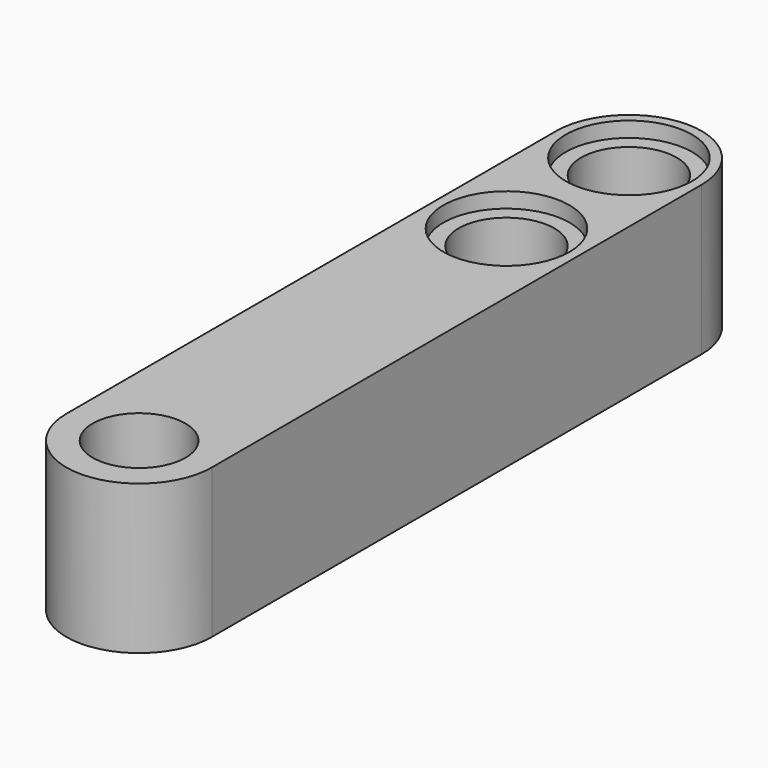
from build123d import *

# Parameters (mm, degrees)
F0_R      = 2.5
F1_DEPTH  = 7.8
F2_R      = 3.3
F3_DEPTH  = 0.8
F4_R      = 3.3
F5_DEPTH  = 0.8
F6_R      = 2.425
F7_DEPTH  = 2.8
F8_R      = 1.75
F9_DEPTH  = 4
F10_R     = 1.15
F11_DEPTH = 5.001
F12_R     = 0.59999
F13_R     = 0.4


# Not quite as in the source:
# - a fillet or chamfer is up to 0.001 mm smaller than in the source, because OpenCascade refuses the exact size


with BuildPart() as f1:
    # F0 (on Top) → F1 (new body)
    with BuildSketch(Plane.XY):
        with BuildLine():
            Line((0, 32), (0, 0))
            ThreePointArc((0, 0), (3.8, -3.8), (7.6, 0))
            Line((7.6, 0), (7.6, 32))
            ThreePointArc((7.6, 32), (3.8, 35.8), (0, 32))
        make_face()
        with Locations((3.8, 24)):
            Circle(F0_R, mode=Mode.SUBTRACT)
        with Locations((3.8, 32)):
            Circle(F0_R, mode=Mode.SUBTRACT)
    extrude(amount=F1_DEPTH)

    # F2 (on face) → F3 (cut)
    with BuildSketch(Plane.XY.offset(7.8)):
        with Locations((3.8, 32)):
            Circle(F2_R)
        with Locations((3.8, 24)):
            Circle(F2_R)
    extrude(amount=-F3_DEPTH, mode=Mode.SUBTRACT)

    # F4 (on face) → F5 (cut)
    with BuildSketch(Plane(origin=(0, 0, 0), x_dir=(1, 0, 0), z_dir=(0, 0, -1))):
        with Locations((3.8, -24)):
            Circle(F4_R)
        with Locations((3.8, -32)):
            Circle(F4_R)
    extrude(amount=-F5_DEPTH, mode=Mode.SUBTRACT)

    # F6 (on face) → F7 (cut)
    with BuildSketch(Plane.XY.offset(7.8)):
        with Locations((3.8, 0)):
            Circle(F6_R)
    extrude(amount=-F7_DEPTH, mode=Mode.SUBTRACT)

    # F8 (on face) → F9 (cut)
    with BuildSketch(Plane(origin=(0, 0, 0), x_dir=(1, 0, 0), z_dir=(0, 0, -1))):
        with Locations((3.8, 0)):
            Circle(F8_R)
    extrude(amount=-F9_DEPTH, mode=Mode.SUBTRACT)

    # F10 (on face) → F11 (cut, through all)
    with BuildSketch(Plane.XY.offset(5)):
        with Locations((3.8, 0)):
            Circle(F10_R)
    extrude(amount=-F11_DEPTH, mode=Mode.SUBTRACT)

    # F12 (radius 0.6 in the source; OpenCascade refuses exactly that, so slightly less here)
    f12_edges = [f1.edges().sort_by_distance(p)[0] for p in [
        (2.05, 0, 4),
    ]]
    fillet(f12_edges, radius=F12_R)

    # F13
    f13_edges = [f1.edges().sort_by_distance(p)[0] for p in [
        (0.5, 24, 0.8),
        (0.5, 32, 0.8),
    ]]
    fillet(f13_edges, radius=F13_R)


solid = f1.part
